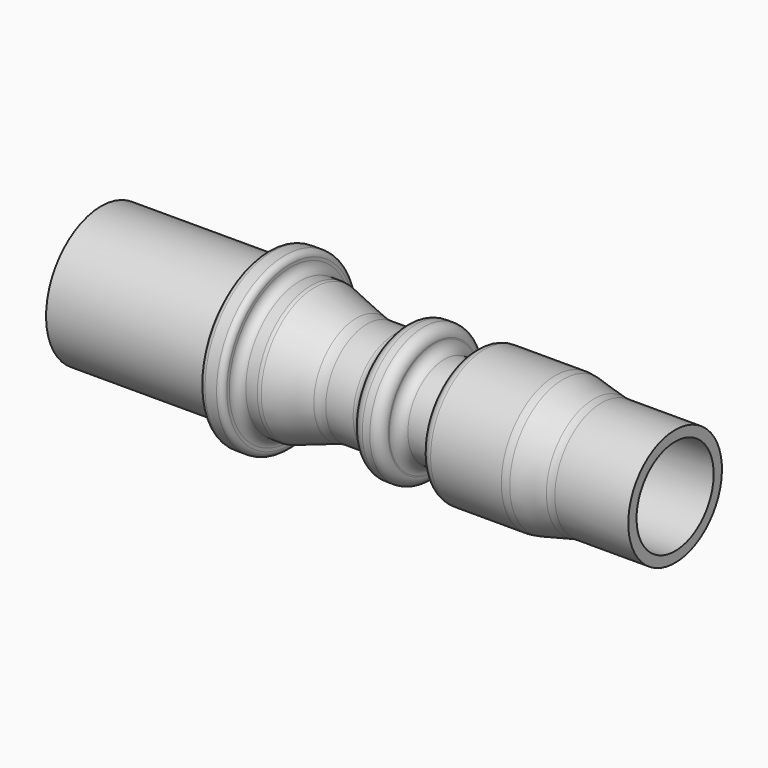
from build123d import *

# Parameters (mm, degrees)
F0_W   = 13.699998
F0_H   = 0.8999982
F0_W_2 = 1.0000234
F0_W_3 = 2.3847298
F0_W_4 = 6.1581792
F0_W_5 = 6.401308


# Not quite as in the source:
# - ends of sketch curves that miss each other by under 0.0002 mm in the source are joined


with BuildPart() as f1:
    # F0 (on Front) → F1 (revolve)
    with BuildSketch(Plane.XZ):
        with Locations((129.4111438469, 114.5151687034)):
            Rectangle(F0_W, F0_H)
        with BuildLine():
            ThreePointArc((137.0611412469, 115.7651662034), (136.8268271404, 115.1994819099), (136.2611428469, 114.9651678034))
            Line((136.2611428469, 114.9651678034), (136.2611428469, 114.0651696034))
            ThreePointArc((136.2611428469, 114.0651696034), (137.3665226637, 114.4736074938), (137.9407496531, 115.502660172))
            Line((137.9407496531, 115.502660172), (138.1667270469, 115.5026572034))
            ThreePointArc((138.1667270469, 115.5026572034), (138.7087012526, 114.390419465), (139.8611356469, 113.9401762034))
            Line((139.8611356469, 113.9401762034), (139.8611356469, 114.8401744034))
            ThreePointArc((139.8611356469, 114.8401744034), (139.2954513533, 115.0744885099), (139.0611372469, 115.6401728034))
            Line((139.0611372469, 115.6401728034), (139.0611372469, 115.9026564034))
            ThreePointArc((139.0611372469, 115.9026564034), (138.9146909303, 116.2562090869), (138.5611382469, 116.4026554034))
            Line((138.5611382469, 116.4026554034), (137.5611402469, 116.4026554034))
            ThreePointArc((137.5611402469, 116.4026554034), (137.2075875634, 116.2562090869), (137.0611412469, 115.9026564034))
            Line((137.0611412469, 115.9026564034), (137.0611412469, 115.7651662034))
        make_face()
        with Locations((140.3611473469, 114.3901753034)):
            Rectangle(F0_W_2, F0_H)
        with BuildLine():
            Line((140.8611590469, 114.8401744034), (140.8611590469, 113.9401762034))
            ThreePointArc((140.8611590469, 113.9401762034), (140.8767965043, 113.9389459834), (140.8920492107, 113.9352855922))
            Line((140.8920492107, 113.9352855922), (141.1701754469, 113.8449043819))
            Line((141.1701754469, 113.8449043819), (141.1701754469, 114.7912286034))
            ThreePointArc((141.1701754469, 114.7912286034), (141.0175935786, 114.8278627086), (140.8611590469, 114.8401744034))
        make_face()
        with BuildLine():
            Line((141.1701754469, 114.7912286034), (141.1701754469, 113.8449043819))
            Line((141.1701754469, 113.8449043819), (144.5213244469, 112.7560536034))
            ThreePointArc((144.5213244469, 112.7560536034), (144.6596565752, 112.7139281426), (144.7994544469, 112.6769569236))
            Line((144.7994544469, 112.6769569236), (144.7994544469, 113.6120082034))
            Line((144.7994544469, 113.6120082034), (141.1701754469, 114.7912286034))
        make_face()
        with BuildLine():
            Line((144.7994544469, 113.6120082034), (144.7994544469, 112.6769569236))
            ThreePointArc((144.7994544469, 112.6769569236), (145.2596214472, 112.5932195337), (145.7265036469, 112.5651726034))
            Line((145.7265036469, 112.5651726034), (145.7265036469, 113.4651708034))
            ThreePointArc((145.7265036469, 113.4651708034), (145.2572000517, 113.5021058881), (144.7994544469, 113.6120082034))
        make_face()
        with BuildLine():
            Line((148.1112334469, 113.4651708034), (148.1112334469, 112.5651726034))
            ThreePointArc((148.1112334469, 112.5651726034), (149.2252053215, 112.9259962262), (149.9160738578, 113.8714208343))
            ThreePointArc((149.9160738578, 113.8714208343), (149.9524213693, 113.9211852123), (150.0110518469, 113.9401762034))
            Line((150.0110518469, 113.9401762034), (150.6611394469, 113.9401762034))
            Line((150.6611394469, 113.9401762034), (150.6611394469, 113.8401764034))
            ThreePointArc((150.6611394469, 113.8401764034), (150.9022932377, 112.9401782034), (151.5611376469, 112.2813337943))
            Line((151.5611376469, 112.2813337943), (151.5611376469, 113.8401764034))
            Line((151.5611376469, 113.8401764034), (151.5611376469, 113.9401762034))
            ThreePointArc((151.5611376469, 113.9401762034), (151.2975342771, 114.5765710337), (150.6611394469, 114.8401744034))
            Line((150.6611394469, 114.8401744034), (150.0110518469, 114.8401744034))
            ThreePointArc((150.0110518469, 114.8401744034), (149.4247506708, 114.6502670965), (149.061135695, 114.1526748904))
            ThreePointArc((149.061135695, 114.1526748904), (148.6975346229, 113.6550781104), (148.1112334469, 113.4651708034))
        make_face()
        with Locations((146.9188685469, 113.0151717034)):
            Rectangle(F0_W_3, F0_H)
        with BuildLine():
            Line((151.5611376469, 113.8401764034), (151.5611376469, 112.2813337943))
            ThreePointArc((151.5611376469, 112.2813337943), (151.9952624974, 112.1015133935), (152.4611358469, 112.0401800034))
            Line((152.4611358469, 112.0401800034), (154.1611578469, 112.0401546034))
            ThreePointArc((154.1611578469, 112.0401546034), (154.6270311963, 112.1015133935), (155.0611560469, 112.2813337943))
            Line((155.0611560469, 112.2813337943), (155.0611560469, 113.8401764034))
            ThreePointArc((155.0611560469, 113.8401764034), (154.7975526771, 113.2037815732), (154.1611578469, 112.9401782034))
            Line((154.1611578469, 112.9401782034), (152.4611358469, 112.9401782034))
            ThreePointArc((152.4611358469, 112.9401782034), (151.8247410166, 113.2037815732), (151.5611376469, 113.8401764034))
        make_face()
        with BuildLine():
            Line((155.0611560469, 113.8401764034), (155.0611560469, 112.2813337943))
            ThreePointArc((155.0611560469, 112.2813337943), (155.720000456, 112.9401782034), (155.9611542469, 113.8401764034))
            Line((155.9611542469, 113.8401764034), (155.9611542469, 113.9401762034))
            Line((155.9611542469, 113.9401762034), (155.9611542469, 114.8401744034))
            ThreePointArc((155.9611542469, 114.8401744034), (155.3247594166, 114.5765710337), (155.0611560469, 113.9401762034))
            Line((155.0611560469, 113.9401762034), (155.0611560469, 113.8401764034))
        make_face()
        with Locations((159.0402438469, 114.3901753034)):
            Rectangle(F0_W_4, F0_H)
        with BuildLine():
            Line((162.1193334469, 114.8401744034), (162.1193334469, 113.9401635034))
            ThreePointArc((162.1193334469, 113.9401635034), (162.3570657373, 113.9266510418), (162.5917415175, 113.8863253226))
            Line((162.5917415175, 113.8863253226), (162.7941860469, 113.8396161217))
            Line((162.7941860469, 113.8396161217), (162.7941860469, 114.7632632034))
            ThreePointArc((162.7941860469, 114.7632632034), (162.4589423593, 114.8208646147), (162.1193334469, 114.8401744034))
        make_face()
        with BuildLine():
            Line((162.7941860469, 114.7632632034), (162.7941860469, 113.8396161217))
            Line((162.7941860469, 113.8396161217), (165.2825478469, 113.2651204034))
            ThreePointArc((165.2825478469, 113.2651204034), (165.3834949467, 113.2432230061), (165.4849858469, 113.2240032152))
            Line((165.4849858469, 113.2240032152), (165.4849858469, 114.1420554034))
            Line((165.4849858469, 114.1420554034), (162.7941860469, 114.7632632034))
        make_face()
        with Locations((169.3604924469, 113.6151705034)):
            Rectangle(F0_W_5, F0_H)
        with BuildLine():
            Line((165.4849858469, 114.1420554034), (165.4849858469, 113.2240032152))
            ThreePointArc((165.4849858469, 113.2240032152), (165.8211323745, 113.1799071954), (166.1598384469, 113.1651714034))
            Line((166.1598384469, 113.1651714034), (166.1598384469, 114.0651696034))
            ThreePointArc((166.1598384469, 114.0651696034), (165.8202295344, 114.0844539922), (165.4849858469, 114.1420554034))
        make_face()
    revolve(axis=Axis((147.5611456469, 0, 108.9651544034), (1, 0, 0)))


solid = f1.part
